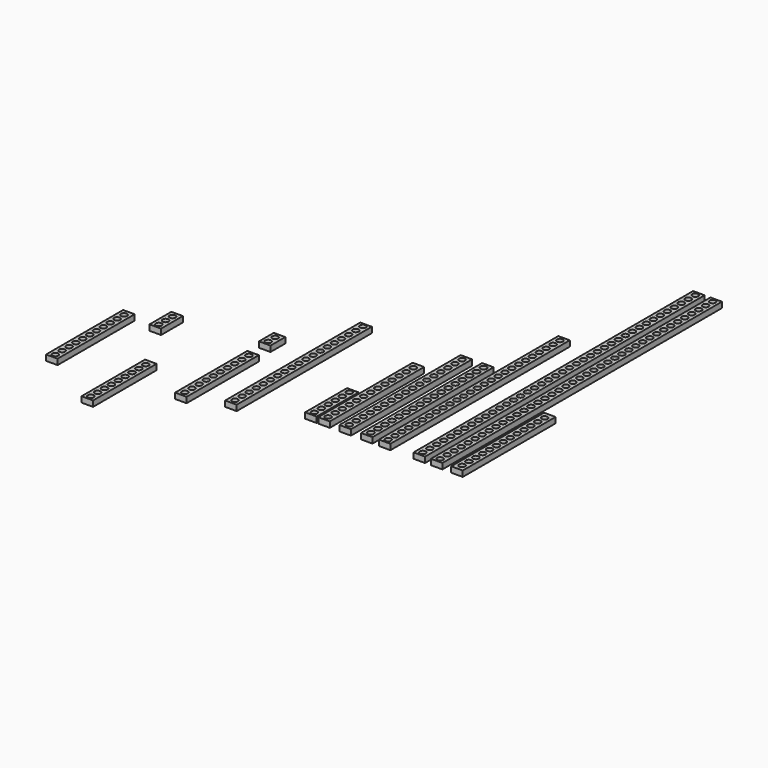
from build123d import *

# Parameters (mm, degrees)
F0_W      = 10.033
F0_H      = 102.87
F0_R      = 2.6035
F1_DEPTH  = 4.953
F2_W      = 10.033
F2_H      = 132.08
F2_R      = 2.6035
F3_DEPTH  = 4.953
F4_W      = 10.033
F4_H      = 132.08
F4_R      = 2.7330632099
F5_DEPTH  = 4.953
F6_W      = 10.033
F6_H      = 195.58
F6_R      = 2.6035
F7_DEPTH  = 4.953
F8_W      = 10.033
F8_H      = 304.8
F8_R      = 2.6035
F9_DEPTH  = 4.953
F10_W     = 10.033
F10_H     = 101.219
F10_R     = 2.6035
F11_DEPTH = 4.953
F12_W     = 10.033
F12_H     = 45.72
F12_R     = 2.6035
F13_DEPTH = 4.953
F14_W     = 10.033
F14_H     = 147.32
F14_R     = 2.6035
F15_DEPTH = 4.953
F16_W     = 10.033
F16_H     = 78.74
F16_R     = 2.6035
F17_DEPTH = 4.953
F18_W     = 10.033
F18_H     = 16.1348620367
F18_R     = 2.6035
F19_DEPTH = 4.953
F21_W     = 10.033
F21_H     = 69.2718740906
F21_R     = 2.6035
F22_DEPTH = 4.953
F20_W     = 10.033
F20_H     = 84.0144696999
F20_R     = 2.6035
F23_W     = 10.033
F23_H     = 23.7891007568
F23_R     = 2.6035
F24_DEPTH = 4.953


# Not quite as in the source:
# - a feature names something its author has since deleted; it is built from what else it names


with BuildPart() as f1:
    # F0 (on Top) → F1 (new body)
    with BuildSketch(Plane.XY):
        with Locations((-58.6581287346, 51.435)):
            Rectangle(F0_W, F0_H)
        with Locations((-58.6581287346, 4.445)):
            Circle(F0_R, mode=Mode.SUBTRACT)
        with Locations((-58.6581287346, 12.192)):
            Circle(F0_R, mode=Mode.SUBTRACT)
        with Locations((-58.6581287346, 19.939)):
            Circle(F0_R, mode=Mode.SUBTRACT)
        with Locations((-58.6581287346, 27.686)):
            Circle(F0_R, mode=Mode.SUBTRACT)
        with Locations((-58.6581287346, 35.433)):
            Circle(F0_R, mode=Mode.SUBTRACT)
        with Locations((-58.6581287346, 43.18)):
            Circle(F0_R, mode=Mode.SUBTRACT)
        with Locations((-58.6581287346, 50.927)):
            Circle(F0_R, mode=Mode.SUBTRACT)
        with Locations((-58.6581287346, 58.674)):
            Circle(F0_R, mode=Mode.SUBTRACT)
        with Locations((-58.6581287346, 66.421)):
            Circle(F0_R, mode=Mode.SUBTRACT)
        with Locations((-58.6581287346, 74.168)):
            Circle(F0_R, mode=Mode.SUBTRACT)
        with Locations((-58.6581287346, 81.915)):
            Circle(F0_R, mode=Mode.SUBTRACT)
        with Locations((-58.6581287346, 89.662)):
            Circle(F0_R, mode=Mode.SUBTRACT)
        with Locations((-58.6581287346, 97.409)):
            Circle(F0_R, mode=Mode.SUBTRACT)
    extrude(amount=F1_DEPTH)


with BuildPart() as f3:
    # F2 (on Top) → F3 (new body)
    with BuildSketch(Plane.XY):
        with Locations((-40.2088483236, 66.04)):
            Rectangle(F2_W, F2_H)
        with Locations((-40.2088483236, 4.445)):
            Circle(F2_R, mode=Mode.SUBTRACT)
        with Locations((-40.2088483236, 12.1285)):
            Circle(F2_R, mode=Mode.SUBTRACT)
        with Locations((-40.2088483236, 19.812)):
            Circle(F2_R, mode=Mode.SUBTRACT)
        with Locations((-40.2088483236, 27.4955)):
            Circle(F2_R, mode=Mode.SUBTRACT)
        with Locations((-40.2088483236, 35.179)):
            Circle(F2_R, mode=Mode.SUBTRACT)
        with Locations((-40.2088483236, 42.8625)):
            Circle(F2_R, mode=Mode.SUBTRACT)
        with Locations((-40.2088483236, 50.546)):
            Circle(F2_R, mode=Mode.SUBTRACT)
        with Locations((-40.2088483236, 58.2295)):
            Circle(F2_R, mode=Mode.SUBTRACT)
        with Locations((-40.2088483236, 65.913)):
            Circle(F2_R, mode=Mode.SUBTRACT)
        with Locations((-40.2088483236, 73.5965)):
            Circle(F2_R, mode=Mode.SUBTRACT)
        with Locations((-40.2088483236, 81.28)):
            Circle(F2_R, mode=Mode.SUBTRACT)
        with Locations((-40.2088483236, 88.9635)):
            Circle(F2_R, mode=Mode.SUBTRACT)
        with Locations((-40.2088483236, 96.647)):
            Circle(F2_R, mode=Mode.SUBTRACT)
        with Locations((-40.2088483236, 104.3305)):
            Circle(F2_R, mode=Mode.SUBTRACT)
        with Locations((-40.2088483236, 112.014)):
            Circle(F2_R, mode=Mode.SUBTRACT)
        with Locations((-40.2088483236, 119.6975)):
            Circle(F2_R, mode=Mode.SUBTRACT)
        with Locations((-40.2088483236, 127.381)):
            Circle(F2_R, mode=Mode.SUBTRACT)
    extrude(amount=F3_DEPTH)


with BuildPart() as f5:
    # F4 (on Top) → F5 (new body)
    with BuildSketch(Plane.XY):
        with Locations((-21.4226992241, 66.04)):
            Rectangle(F4_W, F4_H)
        with Locations((-21.4226992241, 4.445)):
            Circle(F4_R, mode=Mode.SUBTRACT)
        with Locations((-21.4226992241, 12.1285)):
            Circle(F4_R, mode=Mode.SUBTRACT)
        with Locations((-21.4226992241, 19.812)):
            Circle(F4_R, mode=Mode.SUBTRACT)
        with Locations((-21.4226992241, 27.4955)):
            Circle(F4_R, mode=Mode.SUBTRACT)
        with Locations((-21.4226992241, 35.179)):
            Circle(F4_R, mode=Mode.SUBTRACT)
        with Locations((-21.4226992241, 42.8625)):
            Circle(F4_R, mode=Mode.SUBTRACT)
        with Locations((-21.4226992241, 50.546)):
            Circle(F4_R, mode=Mode.SUBTRACT)
        with Locations((-21.4226992241, 58.2295)):
            Circle(F4_R, mode=Mode.SUBTRACT)
        with Locations((-21.4226992241, 65.913)):
            Circle(F4_R, mode=Mode.SUBTRACT)
        with Locations((-21.4226992241, 73.5965)):
            Circle(F4_R, mode=Mode.SUBTRACT)
        with Locations((-21.4226992241, 81.28)):
            Circle(F4_R, mode=Mode.SUBTRACT)
        with Locations((-21.4226992241, 88.9635)):
            Circle(F4_R, mode=Mode.SUBTRACT)
        with Locations((-21.4226992241, 96.647)):
            Circle(F4_R, mode=Mode.SUBTRACT)
        with Locations((-21.4226992241, 104.3305)):
            Circle(F4_R, mode=Mode.SUBTRACT)
        with Locations((-21.4226992241, 112.014)):
            Circle(F4_R, mode=Mode.SUBTRACT)
        with Locations((-21.4226992241, 119.6975)):
            Circle(F4_R, mode=Mode.SUBTRACT)
        with Locations((-21.4226992241, 127.381)):
            Circle(F4_R, mode=Mode.SUBTRACT)
    extrude(amount=F5_DEPTH)


with BuildPart() as f7:
    # F6 (on Top) → F7 (new body)
    with BuildSketch(Plane.XY):
        with Locations((-5.8126096985, 97.79)):
            Rectangle(F6_W, F6_H)
        with Locations((-5.8126096985, 3.81)):
            Circle(F6_R, mode=Mode.SUBTRACT)
        with Locations((-5.8126096985, 11.303)):
            Circle(F6_R, mode=Mode.SUBTRACT)
        with Locations((-5.8126096985, 18.796)):
            Circle(F6_R, mode=Mode.SUBTRACT)
        with Locations((-5.8126096985, 26.289)):
            Circle(F6_R, mode=Mode.SUBTRACT)
        with Locations((-5.8126096985, 33.782)):
            Circle(F6_R, mode=Mode.SUBTRACT)
        with Locations((-5.8126096985, 41.275)):
            Circle(F6_R, mode=Mode.SUBTRACT)
        with Locations((-5.8126096985, 48.768)):
            Circle(F6_R, mode=Mode.SUBTRACT)
        with Locations((-5.8126096985, 56.261)):
            Circle(F6_R, mode=Mode.SUBTRACT)
        with Locations((-5.8126096985, 63.754)):
            Circle(F6_R, mode=Mode.SUBTRACT)
        with Locations((-5.8126096985, 71.247)):
            Circle(F6_R, mode=Mode.SUBTRACT)
        with Locations((-5.8126096985, 78.74)):
            Circle(F6_R, mode=Mode.SUBTRACT)
        with Locations((-5.8126096985, 86.233)):
            Circle(F6_R, mode=Mode.SUBTRACT)
        with Locations((-5.8126096985, 93.726)):
            Circle(F6_R, mode=Mode.SUBTRACT)
        with Locations((-5.8126096985, 101.219)):
            Circle(F6_R, mode=Mode.SUBTRACT)
        with Locations((-5.8126096985, 108.712)):
            Circle(F6_R, mode=Mode.SUBTRACT)
        with Locations((-5.8126096985, 116.205)):
            Circle(F6_R, mode=Mode.SUBTRACT)
        with Locations((-5.8126096985, 123.698)):
            Circle(F6_R, mode=Mode.SUBTRACT)
        with Locations((-5.8126096985, 131.191)):
            Circle(F6_R, mode=Mode.SUBTRACT)
        with Locations((-5.8126096985, 138.684)):
            Circle(F6_R, mode=Mode.SUBTRACT)
        with Locations((-5.8126096985, 146.177)):
            Circle(F6_R, mode=Mode.SUBTRACT)
        with Locations((-5.8126096985, 153.67)):
            Circle(F6_R, mode=Mode.SUBTRACT)
        with Locations((-5.8126096985, 161.163)):
            Circle(F6_R, mode=Mode.SUBTRACT)
        with Locations((-5.8126096985, 168.656)):
            Circle(F6_R, mode=Mode.SUBTRACT)
        with Locations((-5.8126096985, 176.149)):
            Circle(F6_R, mode=Mode.SUBTRACT)
        with Locations((-5.8126096985, 183.642)):
            Circle(F6_R, mode=Mode.SUBTRACT)
        with Locations((-5.8126096985, 191.135)):
            Circle(F6_R, mode=Mode.SUBTRACT)
    extrude(amount=F7_DEPTH)


with BuildPart() as f9:
    # F8 (on Top) → F9 (new body)
    with BuildSketch(Plane.XY):
        with Locations((24.4390162268, 152.4)):
            Rectangle(F8_W, F8_H)
        with Locations((24.4390162268, 3.81)):
            Circle(F8_R, mode=Mode.SUBTRACT)
        with Locations((24.4390162268, 11.43)):
            Circle(F8_R, mode=Mode.SUBTRACT)
        with Locations((24.4390162268, 19.05)):
            Circle(F8_R, mode=Mode.SUBTRACT)
        with Locations((24.4390162268, 26.67)):
            Circle(F8_R, mode=Mode.SUBTRACT)
        with Locations((24.4390162268, 34.29)):
            Circle(F8_R, mode=Mode.SUBTRACT)
        with Locations((24.4390162268, 41.91)):
            Circle(F8_R, mode=Mode.SUBTRACT)
        with Locations((24.4390162268, 49.53)):
            Circle(F8_R, mode=Mode.SUBTRACT)
        with Locations((24.4390162268, 57.15)):
            Circle(F8_R, mode=Mode.SUBTRACT)
        with Locations((24.4390162268, 64.77)):
            Circle(F8_R, mode=Mode.SUBTRACT)
        with Locations((24.4390162268, 72.39)):
            Circle(F8_R, mode=Mode.SUBTRACT)
        with Locations((24.4390162268, 80.01)):
            Circle(F8_R, mode=Mode.SUBTRACT)
        with Locations((24.4390162268, 87.63)):
            Circle(F8_R, mode=Mode.SUBTRACT)
        with Locations((24.4390162268, 95.25)):
            Circle(F8_R, mode=Mode.SUBTRACT)
        with Locations((24.4390162268, 102.87)):
            Circle(F8_R, mode=Mode.SUBTRACT)
        with Locations((24.4390162268, 110.49)):
            Circle(F8_R, mode=Mode.SUBTRACT)
        with Locations((24.4390162268, 118.11)):
            Circle(F8_R, mode=Mode.SUBTRACT)
        with Locations((24.4390162268, 125.73)):
            Circle(F8_R, mode=Mode.SUBTRACT)
        with Locations((24.4390162268, 133.35)):
            Circle(F8_R, mode=Mode.SUBTRACT)
        with Locations((24.4390162268, 140.97)):
            Circle(F8_R, mode=Mode.SUBTRACT)
        with Locations((24.4390162268, 148.59)):
            Circle(F8_R, mode=Mode.SUBTRACT)
        with Locations((24.4390162268, 156.21)):
            Circle(F8_R, mode=Mode.SUBTRACT)
        with Locations((24.4390162268, 163.83)):
            Circle(F8_R, mode=Mode.SUBTRACT)
        with Locations((24.4390162268, 171.45)):
            Circle(F8_R, mode=Mode.SUBTRACT)
        with Locations((24.4390162268, 179.07)):
            Circle(F8_R, mode=Mode.SUBTRACT)
        with Locations((24.4390162268, 186.69)):
            Circle(F8_R, mode=Mode.SUBTRACT)
        with Locations((24.4390162268, 194.31)):
            Circle(F8_R, mode=Mode.SUBTRACT)
        with Locations((24.4390162268, 201.93)):
            Circle(F8_R, mode=Mode.SUBTRACT)
        with Locations((24.4390162268, 209.55)):
            Circle(F8_R, mode=Mode.SUBTRACT)
        with Locations((24.4390162268, 217.17)):
            Circle(F8_R, mode=Mode.SUBTRACT)
        with Locations((24.4390162268, 224.79)):
            Circle(F8_R, mode=Mode.SUBTRACT)
        with Locations((24.4390162268, 232.41)):
            Circle(F8_R, mode=Mode.SUBTRACT)
        with Locations((24.4390162268, 240.03)):
            Circle(F8_R, mode=Mode.SUBTRACT)
        with Locations((24.4390162268, 247.65)):
            Circle(F8_R, mode=Mode.SUBTRACT)
        with Locations((24.4390162268, 255.27)):
            Circle(F8_R, mode=Mode.SUBTRACT)
        with Locations((24.4390162268, 262.89)):
            Circle(F8_R, mode=Mode.SUBTRACT)
        with Locations((24.4390162268, 270.51)):
            Circle(F8_R, mode=Mode.SUBTRACT)
        with Locations((24.4390162268, 278.13)):
            Circle(F8_R, mode=Mode.SUBTRACT)
        with Locations((24.4390162268, 285.75)):
            Circle(F8_R, mode=Mode.SUBTRACT)
        with Locations((24.4390162268, 293.37)):
            Circle(F8_R, mode=Mode.SUBTRACT)
        with Locations((24.4390162268, 300.99)):
            Circle(F8_R, mode=Mode.SUBTRACT)
    extrude(amount=F9_DEPTH)


with BuildPart() as f9b:
    # F8 (on Top) → F9, piece 2 (new body)
    with BuildSketch(Plane.XY):
        with Locations((39.5520162268, 152.4)):
            Rectangle(F8_W, F8_H)
        with Locations((39.5520162268, 3.81)):
            Circle(F8_R, mode=Mode.SUBTRACT)
        with Locations((39.5520162268, 11.43)):
            Circle(F8_R, mode=Mode.SUBTRACT)
        with Locations((39.5520162268, 19.05)):
            Circle(F8_R, mode=Mode.SUBTRACT)
        with Locations((39.5520162268, 26.67)):
            Circle(F8_R, mode=Mode.SUBTRACT)
        with Locations((39.5520162268, 34.29)):
            Circle(F8_R, mode=Mode.SUBTRACT)
        with Locations((39.5520162268, 41.91)):
            Circle(F8_R, mode=Mode.SUBTRACT)
        with Locations((39.5520162268, 49.53)):
            Circle(F8_R, mode=Mode.SUBTRACT)
        with Locations((39.5520162268, 57.15)):
            Circle(F8_R, mode=Mode.SUBTRACT)
        with Locations((39.5520162268, 64.77)):
            Circle(F8_R, mode=Mode.SUBTRACT)
        with Locations((39.5520162268, 72.39)):
            Circle(F8_R, mode=Mode.SUBTRACT)
        with Locations((39.5520162268, 80.01)):
            Circle(F8_R, mode=Mode.SUBTRACT)
        with Locations((39.5520162268, 87.63)):
            Circle(F8_R, mode=Mode.SUBTRACT)
        with Locations((39.5520162268, 95.25)):
            Circle(F8_R, mode=Mode.SUBTRACT)
        with Locations((39.5520162268, 102.87)):
            Circle(F8_R, mode=Mode.SUBTRACT)
        with Locations((39.5520162268, 110.49)):
            Circle(F8_R, mode=Mode.SUBTRACT)
        with Locations((39.5520162268, 118.11)):
            Circle(F8_R, mode=Mode.SUBTRACT)
        with Locations((39.5520162268, 125.73)):
            Circle(F8_R, mode=Mode.SUBTRACT)
        with Locations((39.5520162268, 133.35)):
            Circle(F8_R, mode=Mode.SUBTRACT)
        with Locations((39.5520162268, 140.97)):
            Circle(F8_R, mode=Mode.SUBTRACT)
        with Locations((39.5520162268, 148.59)):
            Circle(F8_R, mode=Mode.SUBTRACT)
        with Locations((39.5520162268, 156.21)):
            Circle(F8_R, mode=Mode.SUBTRACT)
        with Locations((39.5520162268, 163.83)):
            Circle(F8_R, mode=Mode.SUBTRACT)
        with Locations((39.5520162268, 171.45)):
            Circle(F8_R, mode=Mode.SUBTRACT)
        with Locations((39.5520162268, 179.07)):
            Circle(F8_R, mode=Mode.SUBTRACT)
        with Locations((39.5520162268, 186.69)):
            Circle(F8_R, mode=Mode.SUBTRACT)
        with Locations((39.5520162268, 194.31)):
            Circle(F8_R, mode=Mode.SUBTRACT)
        with Locations((39.5520162268, 201.93)):
            Circle(F8_R, mode=Mode.SUBTRACT)
        with Locations((39.5520162268, 209.55)):
            Circle(F8_R, mode=Mode.SUBTRACT)
        with Locations((39.5520162268, 217.17)):
            Circle(F8_R, mode=Mode.SUBTRACT)
        with Locations((39.5520162268, 224.79)):
            Circle(F8_R, mode=Mode.SUBTRACT)
        with Locations((39.5520162268, 232.41)):
            Circle(F8_R, mode=Mode.SUBTRACT)
        with Locations((39.5520162268, 240.03)):
            Circle(F8_R, mode=Mode.SUBTRACT)
        with Locations((39.5520162268, 247.65)):
            Circle(F8_R, mode=Mode.SUBTRACT)
        with Locations((39.5520162268, 255.27)):
            Circle(F8_R, mode=Mode.SUBTRACT)
        with Locations((39.5520162268, 262.89)):
            Circle(F8_R, mode=Mode.SUBTRACT)
        with Locations((39.5520162268, 270.51)):
            Circle(F8_R, mode=Mode.SUBTRACT)
        with Locations((39.5520162268, 278.13)):
            Circle(F8_R, mode=Mode.SUBTRACT)
        with Locations((39.5520162268, 285.75)):
            Circle(F8_R, mode=Mode.SUBTRACT)
        with Locations((39.5520162268, 293.37)):
            Circle(F8_R, mode=Mode.SUBTRACT)
        with Locations((39.5520162268, 300.99)):
            Circle(F8_R, mode=Mode.SUBTRACT)
    extrude(amount=F9_DEPTH)


with BuildPart() as f11:
    # F10 (on Top) → F11 (new body)
    with BuildSketch(Plane.XY):
        with Locations((57.2957600095, 50.6095)):
            Rectangle(F10_W, F10_H)
        with Locations((57.2957600095, 5.588)):
            Circle(F10_R, mode=Mode.SUBTRACT)
        with Locations((57.2957600095, 13.081)):
            Circle(F10_R, mode=Mode.SUBTRACT)
        with Locations((57.2957600095, 20.574)):
            Circle(F10_R, mode=Mode.SUBTRACT)
        with Locations((57.2957600095, 28.067)):
            Circle(F10_R, mode=Mode.SUBTRACT)
        with Locations((57.2957600095, 35.56)):
            Circle(F10_R, mode=Mode.SUBTRACT)
        with Locations((57.2957600095, 43.053)):
            Circle(F10_R, mode=Mode.SUBTRACT)
        with Locations((57.2957600095, 50.546)):
            Circle(F10_R, mode=Mode.SUBTRACT)
        with Locations((57.2957600095, 58.039)):
            Circle(F10_R, mode=Mode.SUBTRACT)
        with Locations((57.2957600095, 65.532)):
            Circle(F10_R, mode=Mode.SUBTRACT)
        with Locations((57.2957600095, 73.025)):
            Circle(F10_R, mode=Mode.SUBTRACT)
        with Locations((57.2957600095, 80.518)):
            Circle(F10_R, mode=Mode.SUBTRACT)
        with Locations((57.2957600095, 88.011)):
            Circle(F10_R, mode=Mode.SUBTRACT)
        with Locations((57.2957600095, 95.504)):
            Circle(F10_R, mode=Mode.SUBTRACT)
    extrude(amount=F11_DEPTH)


with BuildPart() as f13:
    # F12 (on Top) → F13 (new body)
    with BuildSketch(Plane.XY):
        with Locations((-70.1582339964, 22.86)):
            Rectangle(F12_W, F12_H)
        with Locations((-70.1582339964, 3.81)):
            Circle(F12_R, mode=Mode.SUBTRACT)
        with Locations((-70.1582339964, 11.43)):
            Circle(F12_R, mode=Mode.SUBTRACT)
        with Locations((-70.1582339964, 19.05)):
            Circle(F12_R, mode=Mode.SUBTRACT)
        with Locations((-70.1582339964, 26.67)):
            Circle(F12_R, mode=Mode.SUBTRACT)
        with Locations((-70.1582339964, 34.29)):
            Circle(F12_R, mode=Mode.SUBTRACT)
        with Locations((-70.1582339964, 41.91)):
            Circle(F12_R, mode=Mode.SUBTRACT)
    extrude(amount=F13_DEPTH)


with BuildPart() as f15:
    # F14 (on Top) → F15 (new body, through all)
    with BuildSketch(Plane.XY):
        with Locations((-123.5920433497, 53.259813234)):
            Rectangle(F14_W, F14_H)
        with Locations((-123.5920433497, -15.955186766)):
            Circle(F14_R, mode=Mode.SUBTRACT)
        with Locations((-123.5920433497, -8.208186766)):
            Circle(F14_R, mode=Mode.SUBTRACT)
        with Locations((-123.5920433497, -0.461186766)):
            Circle(F14_R, mode=Mode.SUBTRACT)
        with Locations((-123.5920433497, 7.285813234)):
            Circle(F14_R, mode=Mode.SUBTRACT)
        with Locations((-123.5920433497, 15.032813234)):
            Circle(F14_R, mode=Mode.SUBTRACT)
        with Locations((-123.5920433497, 22.779813234)):
            Circle(F14_R, mode=Mode.SUBTRACT)
        with Locations((-123.5920433497, 30.526813234)):
            Circle(F14_R, mode=Mode.SUBTRACT)
        with Locations((-123.5920433497, 38.273813234)):
            Circle(F14_R, mode=Mode.SUBTRACT)
        with Locations((-123.5920433497, 46.020813234)):
            Circle(F14_R, mode=Mode.SUBTRACT)
        with Locations((-123.5920433497, 53.767813234)):
            Circle(F14_R, mode=Mode.SUBTRACT)
        with Locations((-123.5920433497, 61.514813234)):
            Circle(F14_R, mode=Mode.SUBTRACT)
        with Locations((-123.5920433497, 69.261813234)):
            Circle(F14_R, mode=Mode.SUBTRACT)
        with Locations((-123.5920433497, 77.008813234)):
            Circle(F14_R, mode=Mode.SUBTRACT)
        with Locations((-123.5920433497, 84.755813234)):
            Circle(F14_R, mode=Mode.SUBTRACT)
        with Locations((-123.5920433497, 92.502813234)):
            Circle(F14_R, mode=Mode.SUBTRACT)
        with Locations((-123.5920433497, 100.249813234)):
            Circle(F14_R, mode=Mode.SUBTRACT)
        with Locations((-123.5920433497, 107.996813234)):
            Circle(F14_R, mode=Mode.SUBTRACT)
        with Locations((-123.5920433497, 115.743813234)):
            Circle(F14_R, mode=Mode.SUBTRACT)
        with Locations((-123.5920433497, 123.490813234)):
            Circle(F14_R, mode=Mode.SUBTRACT)
    extrude(amount=F15_DEPTH)


with BuildPart() as f17:
    # F16 (on Top) → F17 (new body, through all)
    with BuildSketch(Plane.XY):
        with Locations((-157.5093139505, 6.7757161919)):
            Rectangle(F16_W, F16_H)
        with Locations((-157.5093139505, -28.1492838081)):
            Circle(F16_R, mode=Mode.SUBTRACT)
        with Locations((-157.5093139505, -20.4022838081)):
            Circle(F16_R, mode=Mode.SUBTRACT)
        with Locations((-157.5093139505, -12.6552838081)):
            Circle(F16_R, mode=Mode.SUBTRACT)
        with Locations((-157.5093139505, -4.9082838081)):
            Circle(F16_R, mode=Mode.SUBTRACT)
        with Locations((-157.5093139505, 2.8387161919)):
            Circle(F16_R, mode=Mode.SUBTRACT)
        with Locations((-157.5093139505, 10.5857161919)):
            Circle(F16_R, mode=Mode.SUBTRACT)
        with Locations((-157.5093139505, 18.3327161919)):
            Circle(F16_R, mode=Mode.SUBTRACT)
        with Locations((-157.5093139505, 26.0797161919)):
            Circle(F16_R, mode=Mode.SUBTRACT)
        with Locations((-157.5093139505, 33.8267161919)):
            Circle(F16_R, mode=Mode.SUBTRACT)
        with Locations((-157.5093139505, 41.5737161919)):
            Circle(F16_R, mode=Mode.SUBTRACT)
    extrude(amount=F17_DEPTH)


with BuildPart() as f19:
    # F18 (on Top) → F19 (new body, through all)
    with BuildSketch(Plane.XY):
        with Locations((-160.0993126631, 70.1607306846)):
            Rectangle(F18_W, F18_H)
        with Locations((-160.0993126631, 65.9032996662)):
            Circle(F18_R, mode=Mode.SUBTRACT)
        with Locations((-160.0993126631, 73.5232996662)):
            Circle(F18_R, mode=Mode.SUBTRACT)
    extrude(amount=F19_DEPTH)


with BuildPart() as f22:
    # F21 (on Top) → F22 (new body, through all)
    with BuildSketch(Plane.XY):
        with Locations((-203.9235196208, -41.9711095966)):
            Rectangle(F21_W, F21_H)
        with Locations((-203.9235196208, -72.7970466419)):
            Circle(F21_R, mode=Mode.SUBTRACT)
        with Locations((-203.9235196208, -65.3040466419)):
            Circle(F21_R, mode=Mode.SUBTRACT)
        with Locations((-203.9235196208, -57.8110466419)):
            Circle(F21_R, mode=Mode.SUBTRACT)
        with Locations((-203.9235196208, -50.3180466419)):
            Circle(F21_R, mode=Mode.SUBTRACT)
        with Locations((-203.9235196208, -42.8250466419)):
            Circle(F21_R, mode=Mode.SUBTRACT)
        with Locations((-203.9235196208, -35.3320466419)):
            Circle(F21_R, mode=Mode.SUBTRACT)
        with Locations((-203.9235196208, -27.8390466419)):
            Circle(F21_R, mode=Mode.SUBTRACT)
        with Locations((-203.9235196208, -20.3460466419)):
            Circle(F21_R, mode=Mode.SUBTRACT)
        with Locations((-203.9235196208, -12.8530466419)):
            Circle(F21_R, mode=Mode.SUBTRACT)
    extrude(amount=F22_DEPTH)


with BuildPart() as f22b:
    # F20 (on Top) → F22, piece 2 (new body, through all)
    with BuildSketch(Plane.XY):
        with Locations((-261.2716368531, -1.5854723971)):
            Rectangle(F20_W, F20_H)
        with Locations((-261.2716368531, -39.7827072471)):
            Circle(F20_R, mode=Mode.SUBTRACT)
        with Locations((-261.2716368531, -32.2897072471)):
            Circle(F20_R, mode=Mode.SUBTRACT)
        with Locations((-261.2716368531, -24.7967072471)):
            Circle(F20_R, mode=Mode.SUBTRACT)
        with Locations((-261.2716368531, -17.3037072471)):
            Circle(F20_R, mode=Mode.SUBTRACT)
        with Locations((-261.2716368531, -9.8107072471)):
            Circle(F20_R, mode=Mode.SUBTRACT)
        with Locations((-261.2716368531, -2.3177072471)):
            Circle(F20_R, mode=Mode.SUBTRACT)
        with Locations((-261.2716368531, 5.1752927529)):
            Circle(F20_R, mode=Mode.SUBTRACT)
        with Locations((-261.2716368531, 12.6682927529)):
            Circle(F20_R, mode=Mode.SUBTRACT)
        with Locations((-261.2716368531, 20.1612927529)):
            Circle(F20_R, mode=Mode.SUBTRACT)
        with Locations((-261.2716368531, 27.6542927529)):
            Circle(F20_R, mode=Mode.SUBTRACT)
        with Locations((-261.2716368531, 35.1472927529)):
            Circle(F20_R, mode=Mode.SUBTRACT)
    extrude(amount=F22_DEPTH)


with BuildPart() as f24:
    # F23 (on Top) → F24 (new body, through all)
    with BuildSketch(Plane.XY):
        with Locations((-233.9748615146, 46.9988407276)):
            Rectangle(F23_W, F23_H)
        with Locations((-233.9748615146, 38.9142903492)):
            Circle(F23_R, mode=Mode.SUBTRACT)
        with Locations((-233.9748615146, 46.4072903492)):
            Circle(F23_R, mode=Mode.SUBTRACT)
        with Locations((-233.9748615146, 53.9002903492)):
            Circle(F23_R, mode=Mode.SUBTRACT)
    extrude(amount=F24_DEPTH)


solid = Compound([f1.part, f3.part, f5.part, f7.part, f9.part, f9b.part, f11.part, f13.part, f15.part, f17.part, f19.part, f22.part, f22b.part, f24.part])
